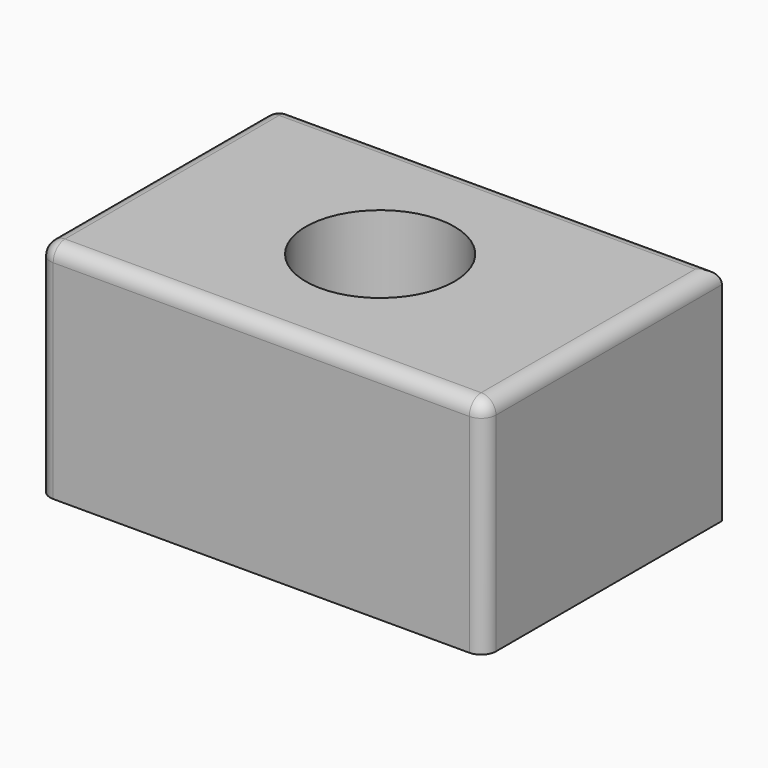
from build123d import *

# Parameters (mm, degrees)
F0_W        = 152.4
F0_H        = 101.6
F0_R        = 25.4
F1_DEPTH    = 76.2
F2_R        = 5.08
F3_R        = 5.08
F4_T1_DEPTH = 83.82
F4_S5_W     = 5.08
F4_S5_H     = 5.08
F4_T6_DEPTH = 5.08


# Not quite as in the source:
# - a fillet or chamfer that OpenCascade refuses, or shapes differently, is made with other operations: its cross-section is extruded or revolved along the edge and cut away or added


with BuildPart() as f1:
    # F0 (on Top) → F1 (new body)
    with BuildSketch(Plane.XY):
        Rectangle(F0_W, F0_H)
        Circle(F0_R, mode=Mode.SUBTRACT)
    extrude(amount=F1_DEPTH)

    # F2
    f2_edges = [f1.edges().sort_by_distance(p)[0] for p in [
        (-76.2, 0, 76.2),
    ]]
    fillet(f2_edges, radius=F2_R)

    # F3
    f3_edges = [f1.edges().sort_by_distance(p)[0] for p in [
        (2.54, 50.8, 76.2),
        (76.2, 0, 76.2),
        (2.54, -50.8, 76.2),
    ]]
    fillet(f3_edges, radius=F3_R)

    # F4: fillet of radius 5.08 on 1 edges, made by hand

    # F4_s2 → F4_t1 (cut)
    with BuildSketch(Plane.XY.offset(-12.7)):
        with BuildLine():
            ThreePointArc((76.2, -45.72), (74.7121024484, -49.3121024484), (71.12, -50.8))
            Line((71.12, -50.8), (76.2, -50.8))
            Line((76.2, -50.8), (76.2, -45.72))
        make_face()
    extrude(amount=F4_T1_DEPTH, mode=Mode.SUBTRACT)


with BuildPart() as f4_tool4:
    # F4_s5 → F4_t6 (new body)
    with BuildSketch(Plane.YZ.offset(71.12)):
        with Locations((-48.26, 73.66)):
            Rectangle(F4_S5_W, F4_S5_H)
    extrude(amount=F4_T6_DEPTH)

    # F4_s7 → F4_t8 (revolve, cut)
    with BuildSketch(Plane(origin=(71.12, -45.72, 71.12), x_dir=(0, 0.7071067812, -0.7071067812), z_dir=(0, -0.7071067812, -0.7071067812))):
        with BuildLine():
            ThreePointArc((0, -5.08), (5.08, 0), (0, 5.08))
            Line((0, 5.08), (0, -5.08))
        make_face()
    revolve(axis=Axis((71.12, -45.72, 71.12), (1, 0, 0)), mode=Mode.SUBTRACT)


with BuildPart() as f1_1:
    add(f1.part)

    # F4_t3: cut F4_tool4
    add(f4_tool4.part, mode=Mode.SUBTRACT)


solid = f1_1.part
